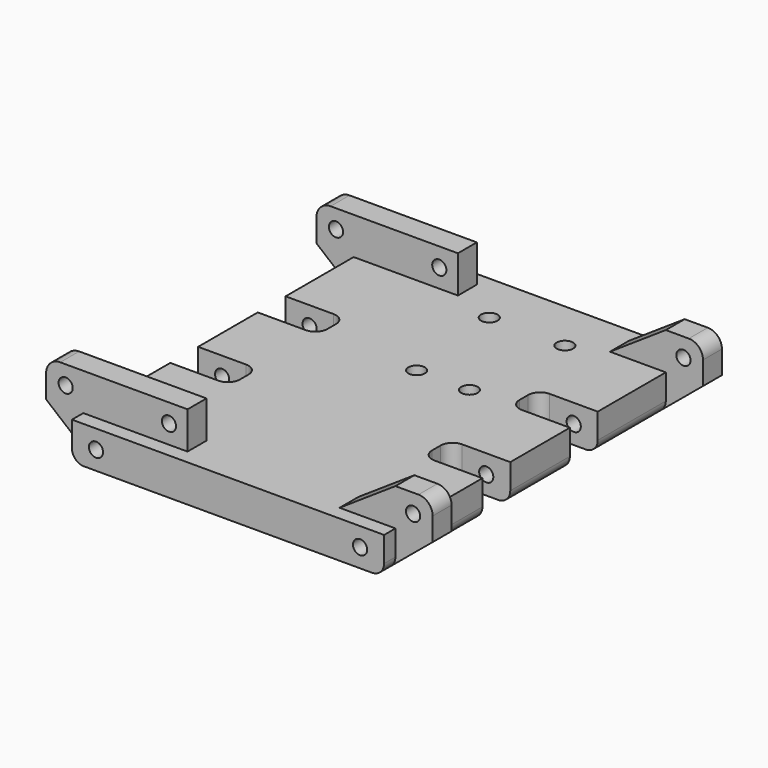
from build123d import *

# Parameters (mm, degrees)
F0_R           = 1.5
F1_DEPTH       = 7.874
F2_R           = 2.54
F3_D           = 3.5
F3_DEPTH       = 10
F3_CSINK_D     = 6
F3_CSINK_ANGLE = 90
F3_TIP         = 1.0515060833
F4_R           = 1.5
F5_DEPTH       = 5
F7_DEPTH       = 76.501
F8_DEPTH       = 3
F10_R          = 3


# Not quite as in the source:
# - a feature names something its author has since deleted; it is built from what else it names


with BuildPart() as f1:
    # F0 (on Top) → F1 (new body)
    with BuildSketch(Plane.XY):
        Polygon((-33.02, -38.25), (0, -38.25), (33.02, -38.25), (33.02, -15.25), (20.32, -15.25), (20.32, -7.884), (33.02, -7.884), (33.02, 0), (33.02, 7.884), (20.32, 7.884), (20.32, 15.25), (33.02, 15.25), (33.02, 38.25), (0, 38.25), (-33.02, 38.25), (-33.02, 15.25), (-20.32, 15.25), (-20.32, 7.884), (-33.02, 7.884), (-33.02, 0), (-33.02, -7.884), (-20.32, -7.884), (-20.32, -15.25), (-33.02, -15.25), align=None)
        with Locations((-1.9812, 30.3125)):
            Circle(F0_R, mode=Mode.SUBTRACT)
        with Locations((0.4318, 8.0875)):
            Circle(F0_R, mode=Mode.SUBTRACT)
        with Locations((11.6078, 8.0875)):
            Circle(F0_R, mode=Mode.SUBTRACT)
        with Locations((14.0208, 30.3125)):
            Circle(F0_R, mode=Mode.SUBTRACT)
    extrude(amount=F1_DEPTH)

    # F2
    f2_edges = [f1.edges().sort_by_distance(p)[0] for p in [
        (20.32, -7.884, 3.937),
        (20.32, -15.25, 3.937),
        (20.32, 7.884, 3.937),
        (20.32, 15.25, 3.937),
        (-20.32, -7.884, 3.937),
        (-20.32, 15.25, 3.937),
        (-20.32, 7.884, 3.937),
        (-20.32, -15.25, 3.937),
        (33.02, -26.75, 0),
        (33.02, 0, 0),
        (33.02, 26.75, 0),
        (-33.02, 26.75, 0),
        (-33.02, 0, 0),
        (-33.02, -26.75, 0),
    ]]
    fillet(f2_edges, radius=F2_R)

    # F3
    with Locations(Plane(origin=(0, 0, 0), x_dir=(1, 0, 0), z_dir=(0, 0, -1))):
        with Locations((0.4318, -8.0875), (11.6078, -8.0875), (14.0208, -30.3125), (-1.9812, -30.3125)):
            CounterSinkHole(F3_D / 2, F3_CSINK_D / 2, depth=F3_DEPTH, counter_sink_angle=F3_CSINK_ANGLE)
            with Locations((0, 0, -(F3_DEPTH + F3_TIP / 2))):  # 118° drill point
                Cone(0, F3_D / 2, F3_TIP, mode=Mode.SUBTRACT)



with BuildPart() as f5:
    # F4 (on face) → F5 (new body)
    with BuildSketch(Plane.XZ.offset(38.25)):
        with BuildLine():
            Line((-33.02, 7.874), (-21.209, 7.874))
            Line((-21.209, 7.874), (-33.02, 15.748))
            Line((-33.02, 15.748), (-40.894, 15.748))
            Line((-40.894, 15.748), (-40.894, 7.874))
            Line((-40.894, 7.874), (-32.10107509, 0.5845676814))
            ThreePointArc((-32.10107509, 0.5845676814), (-32.7788182539, 1.4597062271), (-33.02, 2.54))
            Line((-33.02, 2.54), (-33.02, 7.874))
        make_face()
        with Locations((-36.757, 11.811)):
            Circle(F4_R, mode=Mode.SUBTRACT)
        Polygon((-21.209, 7.874), (-10.963, 7.874), (-10.963, 15.748), (-33.02, 15.748), align=None)
        with Locations((-14.9, 11.811)):
            Circle(F4_R, mode=Mode.SUBTRACT)
    extrude(amount=-F5_DEPTH)


with BuildPart() as f5b:
    # F4 (on face) → F5, piece 2 (new body)
    with BuildSketch(Plane.XZ.offset(38.25)):
        with BuildLine():
            Line((40.894, 15.748), (33.02, 15.748))
            Line((33.02, 15.748), (21.209, 7.874))
            Line((21.209, 7.874), (33.02, 7.874))
            Line((33.02, 7.874), (33.02, 2.54))
            ThreePointArc((33.02, 2.54), (32.7788182539, 1.4597062271), (32.10107509, 0.5845676814))
            Line((32.10107509, 0.5845676814), (40.894, 7.874))
            Line((40.894, 7.874), (40.894, 15.748))
        make_face()
        with Locations((36.757, 11.811)):
            Circle(F4_R, mode=Mode.SUBTRACT)
    extrude(amount=-F5_DEPTH)


with BuildPart() as f1_1:
    add(f1.part)

    add(f5.part)  # F6 merges F5

    add(f5b.part)  # F6 merges F5b
    # F6: F5, F5b across plane
    add(f5.part.mirror(Plane.XZ))
    add(f5b.part.mirror(Plane.XZ))

    # F4 (on face) → F7 (cut, through all)
    with BuildSketch(Plane.XZ.offset(38.25)):
        with Locations((-27.94, 3.937)):
            Circle(F4_R)
        with Locations((27.94, 3.937)):
            Circle(F4_R)
    extrude(amount=-F7_DEPTH, mode=Mode.SUBTRACT)



with BuildPart() as f8:
    # F4 (on face) → F8 (new body)
    with BuildSketch(Plane.XZ.offset(38.25)):
        with BuildLine():
            Line((33.02, 7.874), (21.209, 7.874))
            Line((21.209, 7.874), (-10.963, 7.874))
            Line((-10.963, 7.874), (-21.209, 7.874))
            Line((-21.209, 7.874), (-33.02, 7.874))
            Line((-33.02, 7.874), (-33.02, 2.54))
            ThreePointArc((-33.02, 2.54), (-32.7788182539, 1.4597062271), (-32.10107509, 0.5845676814))
            ThreePointArc((-32.10107509, 0.5845676814), (-31.3416269236, 0.1506069715), (-30.48, 0))
            Line((-30.48, 0), (30.48, 0))
            ThreePointArc((30.48, 0), (31.3416269236, 0.1506069715), (32.10107509, 0.5845676814))
            ThreePointArc((32.10107509, 0.5845676814), (32.7788182539, 1.4597062271), (33.02, 2.54))
            Line((33.02, 2.54), (33.02, 7.874))
        make_face()
        with Locations((-27.94, 3.937)):
            Circle(F4_R, mode=Mode.SUBTRACT)
        with Locations((27.94, 3.937)):
            Circle(F4_R, mode=Mode.SUBTRACT)
    extrude(amount=F8_DEPTH)


with BuildPart() as f1_2:
    add(f1_1.part)

    add(f8.part)  # F9 merges F8
    # F9: F8 across plane
    add(f8.part.mirror(Plane.XZ))

    # F10
    f10_edges = [f1_2.edges().sort_by_distance(p)[0] for p in [
        (-40.894, -35.75, 15.748),
        (40.894, 35.75, 15.748),
        (40.894, -35.75, 15.748),
        (-40.894, 35.75, 15.748),
    ]]
    fillet(f10_edges, radius=F10_R)


solid = f1_2.part
